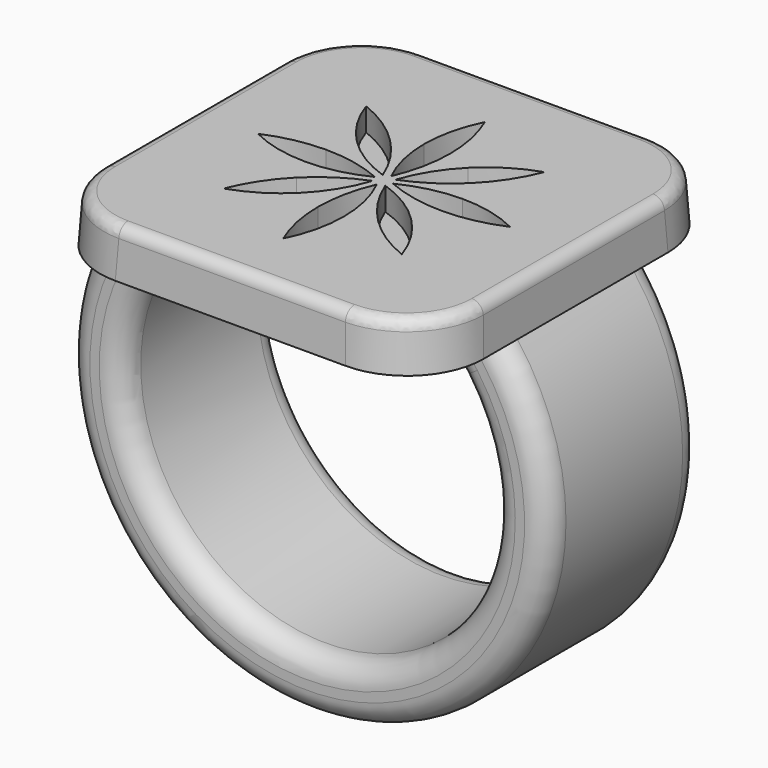
from build123d import *

# Parameters (mm, degrees)
F0_W          = 25.4
F0_H          = 25.4
F1_DEPTH      = 3.175
F1_TAPER      = 3
F3_W          = 5.08
F3_H          = 12.7
F6_DEPTH      = 6.35
F6_DEPTH_BACK = 6.35
F7_R          = 5.08
F8_R          = 1.524
F9_R          = 0.762
F11_DEPTH     = 1.524


# Not quite as in the source:
# - ends of sketch curves that miss each other by under 0.0002 mm in the source are joined


with BuildPart() as f1:
    # F0 (on Top) → F1 (new body)
    with BuildSketch(Plane.XY):
        Rectangle(F0_W, F0_H)
    extrude(amount=F1_DEPTH, taper=F1_TAPER)

    # F4: sweep along a path in F2
    with BuildLine(Plane.XZ) as f4_path:
        ThreePointArc((-10.16, 0), (0, -23.5582897328), (10.16, 0))
    # F3 (on face) → F4 (sweep)
    with BuildSketch(Plane(origin=(0, 0, 0), x_dir=(1, 0, 0), z_dir=(0, 0, -1))):
        with Locations((-10.16, 0)):
            Rectangle(F3_W, F3_H)
    sweep(path=f4_path.line)

    # F5 (on Front) → F6 (join, two sides)
    with BuildSketch(Plane.XZ) as f6_sk:
        with BuildLine():
            ThreePointArc((7.62, 0), (8.9072265211, -1.1822790439), (10.0130578512, -2.535746045))
            Line((10.0130578512, -2.535746045), (10.16, 0))
            Line((10.16, 0), (7.62, 0))
        make_face()
    extrude(amount=F6_DEPTH)
    extrude(f6_sk.sketch, amount=-F6_DEPTH_BACK)

    # F7
    f7_edges = [f1.edges().sort_by_distance(p)[0] for p in [
        (-12.616803, 12.616803, 1.5875),
        (-12.616803, -12.616803, 1.5875),
        (12.616803, -12.616803, 1.5875),
        (12.616803, 12.616803, 1.5875),
    ]]
    fillet(f7_edges, radius=F7_R)

    # F8
    f8_edges = [f1.edges().sort_by_distance(p)[0] for p in [
        (-1.743325, -6.35, -21.711017),
        (8.907227, -6.35, -1.182279),
        (-1.743325, 6.35, -21.711017),
        (0, -6.35, -25.501344),
        (0, 6.35, -25.501344),
        (8.907227, 6.35, -1.182279),
    ]]
    fillet(f8_edges, radius=F8_R)

    # F9
    f9_edges = [f1.edges().sort_by_distance(p)[0] for p in [
        (12.533605, 0, 3.175),
        (11.048589, -11.048589, 3.175),
        (11.048589, 11.048589, 3.175),
        (0, -12.533605, 3.175),
        (0, 12.533605, 3.175),
        (-11.048589, -11.048589, 3.175),
        (-11.048589, 11.048589, 3.175),
        (-12.533605, 0, 3.175),
    ]]
    fillet(f9_edges, radius=F9_R)

    # F10 (on face) → F11 (cut)
    with BuildSketch(Plane.XY.offset(3.175)):
        with BuildLine():
            ThreePointArc((-0.9155427616, 4.4694347941), (-0.6833212656, 2.4793847644), (-1.9106e-05, 0.5959506396))
            ThreePointArc((-1.9106e-05, 0.5959506396), (0.6027711391, 2.4909604876), (0.8062465423, 4.4690791999))
            ThreePointArc((0.8062465423, 4.4690791999), (0.6018941572, 6.4474337167), (-0.0016602711, 8.3425243592))
            ThreePointArc((-0.0016602711, 8.3425243592), (-0.6841876238, 6.4592135153), (-0.9155427616, 4.4694347941))
        make_face()
        with BuildLine():
            ThreePointArc((-3.8077433876, 2.5129958106), (-2.2363648369, 1.2700255802), (-0.4214138117, 0.4214041575))
            ThreePointArc((-0.4214138117, 0.4214041575), (-1.3351477858, 2.1876037686), (-2.5900078566, 3.7302233456))
            ThreePointArc((-2.5900078566, 3.7302233456), (-4.1334248315, 4.984630209), (-5.9002408115, 5.8978835339))
            ThreePointArc((-5.9002408115, 5.8978835339), (-5.0511449244, 4.0835594737), (-3.8077433876, 2.5129958106))
        make_face()
        with BuildLine():
            ThreePointArc((2.5129831047, 3.8077560876), (1.2700048982, 2.2363724755), (0.4213787575, 0.4214138117))
            ThreePointArc((0.4213787575, 0.4214138117), (2.1875938836, 1.3351413072), (3.7302233456, 2.5900078566))
            ThreePointArc((3.7302233456, 2.5900078566), (4.984630209, 4.1334248315), (5.8978835339, 5.9002408115))
            ThreePointArc((5.8978835339, 5.9002408115), (4.0835594737, 5.0511449244), (2.5129831047, 3.8077560876))
        make_face()
        with BuildLine():
            ThreePointArc((-4.4694348001, -0.9155173616), (-2.4793902981, -0.6832971735), (-0.5959608043, 1.2077e-06))
            ThreePointArc((-0.5959608043, 1.2077e-06), (-2.4909555235, 0.6027955057), (-4.4690791999, 0.8062719423))
            ThreePointArc((-4.4690791999, 0.8062719423), (-6.4474386841, 0.6019185211), (-8.3425336625, -0.0016389259))
            ThreePointArc((-8.3425336625, -0.0016389259), (-6.4592135153, -0.6841876238), (-4.4694348001, -0.9155173616))
        make_face()
        with BuildLine():
            ThreePointArc((-2.5129958106, -3.8077433876), (-1.2700192482, -2.2363545852), (-0.4213965439, -0.4213909469))
            ThreePointArc((-0.4213965439, -0.4213909469), (-2.1876037686, -1.3351223858), (-3.7302233456, -2.5899824566))
            ThreePointArc((-3.7302233456, -2.5899824566), (-4.9846188126, -4.1334074282), (-5.8978748887, -5.9002188082))
            ThreePointArc((-5.8978748887, -5.9002188082), (-4.0835560578, -5.0511428128), (-2.5129958106, -3.8077433876))
        make_face()
        with BuildLine():
            ThreePointArc((0.9155173616, -4.4694348001), (0.6832945611, -2.4793792452), (-1.13725e-05, -0.5959404907))
            ThreePointArc((-1.13725e-05, -0.5959404907), (-0.6027905445, -2.4909316905), (-0.8062719482, -4.4690537999))
            ThreePointArc((-0.8062719482, -4.4690537999), (-0.601916144, -6.447424681), (0.0016482293, -8.3425296076))
            ThreePointArc((0.0016482293, -8.3425296076), (0.6841820987, -6.4592115314), (0.9155173616, -4.4694348001))
        make_face()
        with BuildLine():
            ThreePointArc((3.8077560876, -2.5129831047), (2.2363622238, -1.2699985662), (0.4213909469, -0.4213711439))
            ThreePointArc((0.4213909469, -0.4213711439), (1.3351159072, -2.1875938836), (2.5899824566, -3.7302233456))
            ThreePointArc((2.5899824566, -3.7302233456), (4.1334074282, -4.9846188126), (5.9002188082, -5.8978748887))
            ThreePointArc((5.9002188082, -5.8978748887), (5.0511428128, -4.0835560578), (3.8077560876, -2.5129831047))
        make_face()
        with BuildLine():
            ThreePointArc((4.4694347941, 0.9155427616), (2.4793737115, 0.6833186532), (0.5959303259, 8.9412e-06))
            ThreePointArc((0.5959303259, 8.9412e-06), (2.4909366547, -0.6027661778), (4.4690537999, -0.8062465482))
            ThreePointArc((4.4690537999, -0.8062465482), (6.4474197136, -0.6018917801), (8.3425203043, 0.0016695744))
            ThreePointArc((8.3425203043, 0.0016695744), (6.4592115314, 0.6841820987), (4.4694347941, 0.9155427616))
        make_face()
    extrude(amount=-F11_DEPTH, mode=Mode.SUBTRACT)


solid = f1.part
